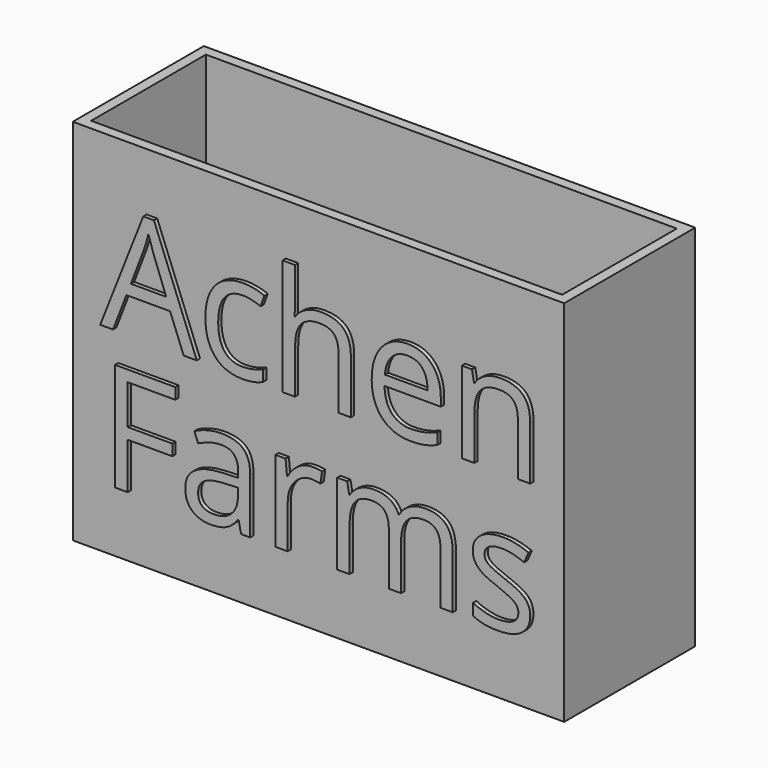
from build123d import *

# Parameters (mm, degrees)
F0_W           = 152.4
F0_H           = 50.8
F1_DEPTH       = 114.3
F2_T           = -3.175
F3_TEXT_SIZE   = 47.337068057
F3_TEXT_SIZE_2 = 46.9258261396
F4_DEPTH       = 1.27


# Not quite as in the source:
# - Text() gives the source's letters only with a copy of the font that has no kerning and outlines rounded to 1/6400 em; it was checked with that copy


with BuildPart() as f1:
    # F0 (on Top) → F1 (new body)
    with BuildSketch(Plane.XY):
        Rectangle(F0_W, F0_H)
    extrude(amount=-F1_DEPTH)

    # F2
    f2_openings = [f1.faces().sort_by_distance(p)[0] for p in [
        (0, 0, 0),
    ]]
    offset(amount=F2_T, openings=f2_openings)


with BuildPart() as f4:
    # F3 (on face) → F4 (new body)
    with BuildSketch(Plane.XZ.offset(25.4)):
        with Locations((-66.675, -51.8201710953)):
            Text('Achen', F3_TEXT_SIZE, font='Open Sans', text_align=(TextAlign.LEFT, TextAlign.BOTTOM))
        with Locations((-66.675, -94.7677343848)):
            Text('Farms', F3_TEXT_SIZE_2, font='Open Sans', text_align=(TextAlign.LEFT, TextAlign.BOTTOM))
    extrude(amount=F4_DEPTH)


solid = Compound([f1.part, f4.part])
